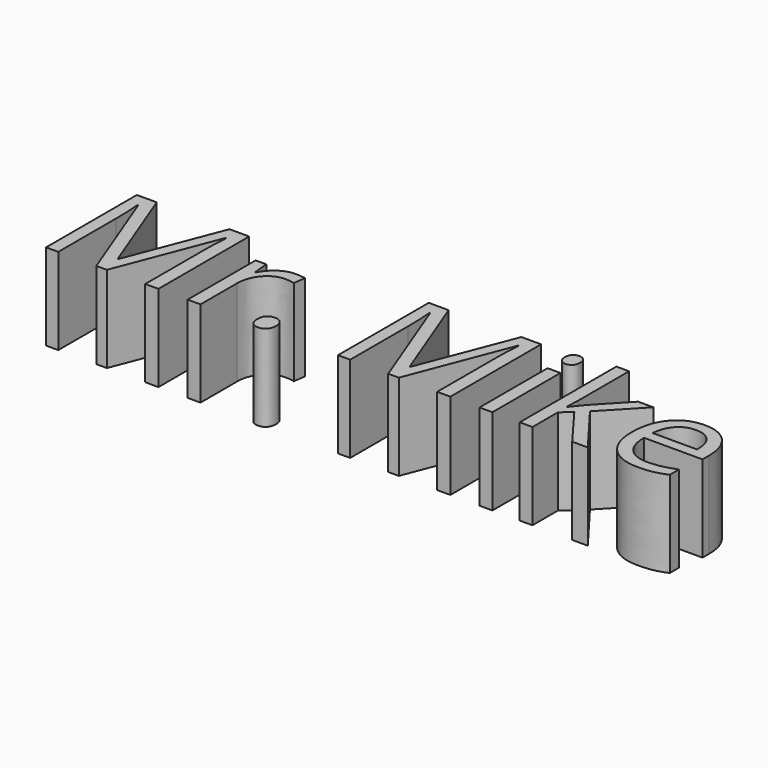
from build123d import *

# Parameters (mm, degrees)
F0_TEXT_SIZE = 46.6560065332
F1_DEPTH     = 25.4


# Not quite as in the source:
# - Text() gives the source's letters only with a copy of the font that has no kerning and outlines rounded to 1/6400 em; it was checked with that copy


with BuildPart() as f1:
    # F0 (on Top) → F1 (new body)
    with BuildSketch(Plane.XY):
        with Locations((-151.7738255498, 0.0601257198)):
            Text('Mr. Mike', F0_TEXT_SIZE, font='Open Sans', text_align=(TextAlign.LEFT, TextAlign.BOTTOM))
    extrude(amount=F1_DEPTH)


solid = f1.part
